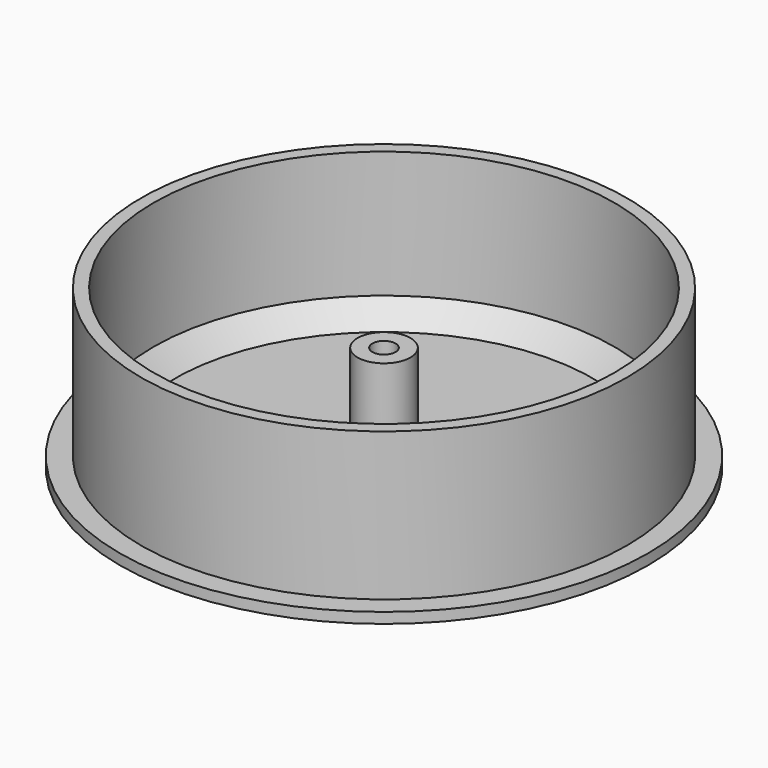
from build123d import *

# Parameters (mm, degrees)
F0_R     = 50
F0_R_2   = 46
F0_R_3   = 43.6
F0_R_4   = 5
F1_DEPTH = 2
F2_DEPTH = 30
F0_R_5   = 2.2
F3_DEPTH = 20
F4_SIZE  = 4


with BuildPart() as f1:
    # F0 (on Top) → F1 (new body)
    with BuildSketch(Plane.XY):
        Circle(F0_R)
        Circle(F0_R_2, mode=Mode.SUBTRACT)
        Circle(F0_R_2)
        Circle(F0_R_3, mode=Mode.SUBTRACT)
        Circle(F0_R_3)
        Circle(F0_R_4, mode=Mode.SUBTRACT)
    extrude(amount=F1_DEPTH)

    # F0 (on Top) → F2 (join)
    with BuildSketch(Plane.XY):
        Circle(F0_R_2)
        Circle(F0_R_3, mode=Mode.SUBTRACT)
    extrude(amount=F2_DEPTH)

    # F0 (on Top) → F3 (join)
    with BuildSketch(Plane.XY):
        Circle(F0_R_4)
        Circle(F0_R_5, mode=Mode.SUBTRACT)
    extrude(amount=F3_DEPTH)

    # F4
    f4_edges = [f1.edges().sort_by_distance(p)[0] for p in [
        (-5, 0, 2),
        (-43.6, 0, 2),
    ]]
    chamfer(f4_edges, length=F4_SIZE)


solid = f1.part
